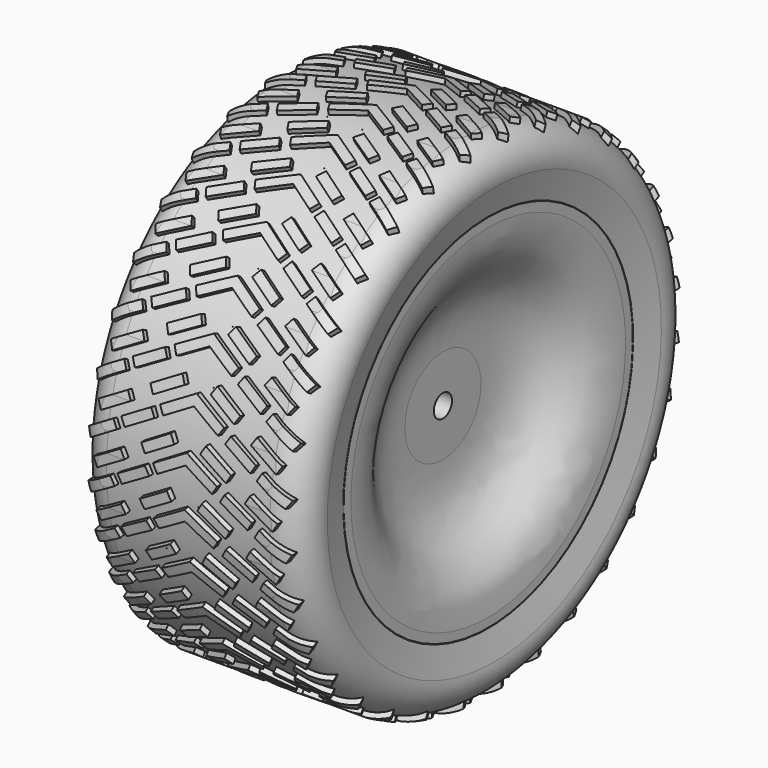
from build123d import *

# Parameters (mm, degrees)
F3_DEPTH        = 4
F8_DEPTH        = 5
F8_COPIES_COUNT = 32


# Not quite as in the source:
# - a pattern or mirror of a feature is missing from the dataset's text; its kind, count and spacing are read off the source's solid


with BuildPart() as f1:
    # F0 (on Front) → F1 (revolve)
    with BuildSketch(Plane.XZ):
        Polygon((3, 2.5), (23, 2.5), (23, 39.9000011384), (20.9000011384, 39.9000011384), (20.9000011384, 41.9000011384), (19.0999988616, 41.9000011384), (19.0999988616, 39.9000011384), (-19.0999988616, 39.9000011384), (-19.0999988616, 41.9000011384), (-20.9000011384, 41.9000011384), (-20.9000011384, 39.9000011384), (-23, 39.9000011384), (-23, 36), (3, 36), align=None)
    revolve(axis=Axis((14.2499990779, 0, 0), (1, 0, 0)))

    # F2 (on face) → F3 (cut)
    with BuildSketch(Plane(origin=(3, 0, 0), x_dir=(0, -1, 0), z_dir=(-1, 0, 0))):
        Polygon((8.5, -4.9074772881), (8.5, 4.9074772881), (0, 9.8149545762), (-8.5, 4.9074772881), (-8.5, -4.9074772881), (0, -9.8149545762), align=None)
    extrude(amount=-F3_DEPTH, mode=Mode.SUBTRACT)

    # F4 (on Front) → F5 (revolve, cut)
    with BuildSketch(Plane.XZ):
        with BuildLine():
            Line((13, 10.5), (13, 0))
            Line((13, 0), (24, 0))
            Line((24, 0), (24, 39.9000011384))
            Line((24, 39.9000011384), (23, 39.9000011384))
            Line((23, 39.9000011384), (23, 37.9000011384))
            add(Edge.make_bspline(
                [(23, 37.9000011384), (23, 24.0901117427), (13, 27.9946189986), (13, 10.5)],
                knots=[0, 0, 0, 0, 29.167791524, 29.167791524, 29.167791524, 29.167791524], degree=3))
        make_face()
    revolve(axis=Axis((22.6738695055, 0, 0), (1, 0, 0)), mode=Mode.SUBTRACT)


with BuildPart() as f1b:
    # F0 (on Front) → F1, piece 2 (revolve)
    with BuildSketch(Plane.XZ):
        with BuildLine():
            Line((-24.346998799, 46.0979991994), (-23, 40))
            Line((-23, 40), (-21, 40))
            Line((-21, 40), (-21, 42))
            Line((-21, 42), (-19, 42))
            Line((-19, 42), (-19, 40))
            Line((-19, 40), (19, 40))
            Line((19, 40), (19, 42))
            Line((19, 42), (21, 42))
            Line((21, 42), (21, 40))
            Line((21, 40), (23, 40))
            Line((23, 40), (24.346998799, 46.0979991994))
            ThreePointArc((24.346998799, 46.0979991994), (23.067692039, 51.5704419168), (18, 54))
            Line((18, 54), (-18, 54))
            ThreePointArc((-18, 54), (-23.067692039, 51.5704419168), (-24.346998799, 46.0979991994))
        make_face()
    revolve(axis=Axis((14.2499990779, 0, 0), (1, 0, 0)))

    # F7 (on offset) → F8 (join)
    with BuildSketch(Plane.XY.offset(55)):
        Polygon((15.4378221735, -2.5), (21.5, -6), (22.5, -4.2679491924), (16.4378221735, -0.7679491924), align=None)
        Polygon((-16.4378221735, -0.7679491924), (-22.5, -4.2679491924), (-21.5, -6), (-15.4378221735, -2.5), align=None)
        Polygon((-8.7942286341, 3.6450815951), (-14.8564064606, 0.1450815951), (-13.8564064606, -1.5869692124), (-7.7942286341, 1.9130307876), align=None)
        Polygon((14.8564064606, 0.1450815951), (8.7942286341, 3.6450815951), (7.7942286341, 1.9130307876), (13.8564064606, -1.5869692124), align=None)
        Polygon((6.0621778265, 2.9130307876), (7.0621778265, 4.6450815951), (0, 8.7224318643), (-7.0621778265, 4.6450815951), (-6.0621778265, 2.9130307876), (0, 6.4130307876), align=None)
        Polygon((-14.2583302492, 5.1091832103), (-20.3205080757, 1.6091832103), (-19.3205080757, -0.1228675973), (-13.2583302492, 3.3771324027), align=None)
        Polygon((-9.9282032303, 7.6091832103), (-8.9282032303, 5.8771324027), (-2.8660254038, 9.3771324027), (-3.8660254038, 11.1091832103), align=None)
        Polygon((9.9282032303, 7.6091832103), (3.8660254038, 11.1091832103), (2.8660254038, 9.3771324027), (8.9282032303, 5.8771324027), align=None)
        Polygon((14.2583302492, 5.1091832103), (13.2583302492, 3.3771324027), (19.3205080757, -0.1228675973), (20.3205080757, 1.6091832103), align=None)
    f8 = extrude(amount=-F8_DEPTH)

    # F8_copies: F8 ×32 about axis
    f8_copies_axis = Axis((0, 0, 0), (1, 0, 0))
    for i in range(1, F8_COPIES_COUNT):
        add(f8.rotate(f8_copies_axis, i * 360 / F8_COPIES_COUNT))

    # F9 (on Front) → F10 (revolve, cut)
    with BuildSketch(Plane.XZ):
        with BuildLine():
            ThreePointArc((-25.6, 47.5), (-23.374011537, 52.874011537), (-18, 55.1))
            Line((-18, 55.1), (18, 55.1))
            ThreePointArc((18, 55.1), (23.374011537, 52.874011537), (25.6, 47.5))
            Line((25.6, 47.5), (29, 47.5))
            Line((29, 47.5), (29, 56.1))
            Line((29, 56.1), (-29, 56.1))
            Line((-29, 56.1), (-29, 47.5))
            Line((-29, 47.5), (-25.6, 47.5))
        make_face()
    revolve(axis=Axis((30.0784315914, 0, 0), (1, 0, 0)), mode=Mode.SUBTRACT)


solid = Compound([f1.part, f1b.part])
